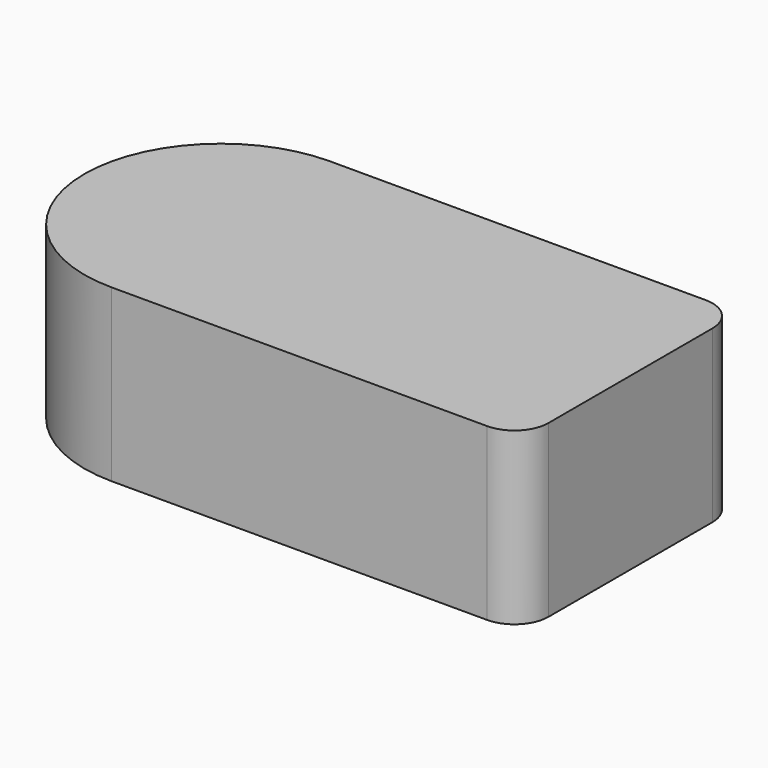
from build123d import *

# Parameters (mm, degrees)
F0_W     = 80
F0_H     = 40
F1_DEPTH = 25
F2_R     = 19.99999
F3_R     = 5


# Not quite as in the source:
# - a fillet or chamfer is up to 0.001 mm smaller than in the source, because OpenCascade refuses the exact size


with BuildPart() as f1:
    # F0 (on Top) → F1 (new body)
    with BuildSketch(Plane.XY):
        with Locations((40, 20)):
            Rectangle(F0_W, F0_H)
    extrude(amount=F1_DEPTH)

    # F2 (radius 20 in the source; OpenCascade refuses exactly that, so slightly less here)
    f2_edges = [f1.edges().sort_by_distance(p)[0] for p in [
        (0, 40, 12.5),
        (0, 0, 12.5),
    ]]
    fillet(f2_edges, radius=F2_R)

    # F3
    f3_edges = [f1.edges().sort_by_distance(p)[0] for p in [
        (80, 40, 12.5),
        (80, 0, 12.5),
    ]]
    fillet(f3_edges, radius=F3_R)


solid = f1.part
